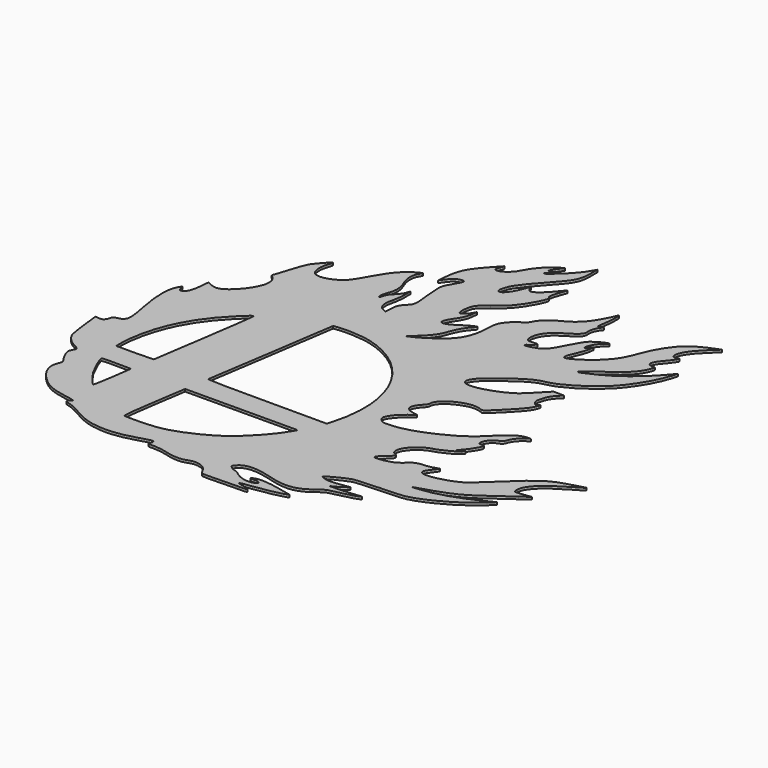
from build123d import *

# Parameters (mm, degrees)
F1_DEPTH = 0.4


# Not quite as in the source:
# - ends of sketch curves that miss each other by under 0.0002 mm in the source are joined


with BuildPart() as f1:
    # F0 (on Top) → F1 (new body)
    with BuildSketch(Plane.XY):
        with BuildLine():
            add(Edge.make_bspline(
                [(-1.4960361405, -38.6585897683), (-1.616879416, -38.6031296058), (-1.8647027683, -38.265785706), (-2.0467534003, -37.9089393314)],
                knots=[0, 0, 0, 0, 1, 1, 1, 1], degree=3))
            add(Edge.make_bspline(
                [(0.6166918414, -38.6753123078), (-0.4244712896, -38.7216066193), (-1.3752026214, -38.7140941599), (-1.4960361405, -38.6585897683)],
                knots=[0, 0, 0, 0, 1, 1, 1, 1], degree=3))
            add(Edge.make_bspline(
                [(4.3166854176, -38.5834606212), (3.3228507809, -38.5878510196), (1.6578504194, -38.6290231997), (0.6166918414, -38.6753123078)],
                knots=[0, 0, 0, 0, 1, 1, 1, 1], degree=3))
            add(Edge.make_bspline(
                [(5.6934265327, -38.3445448994), (6.0777086692, -38.5510887507), (5.9306739032, -38.5766063964), (4.3166854176, -38.5834606212)],
                knots=[0, 0, 0, 0, 1, 1, 1, 1], degree=3))
            add(Edge.make_bspline(
                [(4.5029020498, -37.9872393216), (4.9210631017, -38.0565737933), (5.4567990215, -38.2173599373), (5.6934265327, -38.3445448994)],
                knots=[0, 0, 0, 0, 1, 1, 1, 1], degree=3))
            add(Edge.make_bspline(
                [(5.8868336618, -37.4158195449), (3.8808118727, -37.6312027316), (3.4438156867, -37.811633144), (4.5029020498, -37.9872393216)],
                knots=[0, 0, 0, 0, 1, 1, 1, 1], degree=3))
            add(Edge.make_bspline(
                [(11.0283023377, -36.219943329), (11.677959013, -36.3096681115), (7.8099744864, -37.2093342322), (5.8868336618, -37.4158195449)],
                knots=[0, 0, 0, 0, 1, 1, 1, 1], degree=3))
            add(Edge.make_bspline(
                [(8.8203417373, -35.7401651502), (9.7980932067, -35.9713635274), (10.791674176, -36.1872638054), (11.0283023377, -36.219943329)],
                knots=[0, 0, 0, 0, 1, 1, 1, 1], degree=3))
            add(Edge.make_bspline(
                [(4.4887792766, -35.5779448093), (5.138255783, -35.2066686588), (6.8325007504, -35.2701193462), (8.8203417373, -35.7401651502)],
                knots=[0, 0, 0, 0, 1, 1, 1, 1], degree=3))
            add(Edge.make_bspline(
                [(4.865826687, -35.829982944), (4.0790868153, -35.8240315151), (4.069491681, -35.8176410464), (4.4887792766, -35.5779448093)],
                knots=[0, 0, 0, 0, 1, 1, 1, 1], degree=3))
            add(Edge.make_bspline(
                [(4.8935349788, -36.6414118144), (6.1954201273, -36.4667910373), (6.1740190492, -35.8398662185), (4.865826687, -35.829982944)],
                knots=[0, 0, 0, 0, 1, 1, 1, 1], degree=3))
            add(Edge.make_bspline(
                [(2.1650389935, -35.8356859089), (2.9463445277, -36.4565955566), (3.9849176489, -36.7632840692), (4.8935349788, -36.6414118144)],
                knots=[0, 0, 0, 0, 1, 1, 1, 1], degree=3))
            add(Edge.make_bspline(
                [(1.2144253893, -35.3198043461), (1.380226344, -35.3198043461), (1.8080020431, -35.5519536511), (2.1650389935, -35.8356859089)],
                knots=[0, 0, 0, 0, 1, 1, 1, 1], degree=3))
            add(Edge.make_bspline(
                [(0.5066931751, -34.9898610318), (0.7301449383, -35.1713308303), (1.0486244347, -35.3198043461), (1.2144253893, -35.3198043461)],
                knots=[0, 0, 0, 0, 1, 1, 1, 1], degree=3))
            Line((0.5066931751, -34.9898610318), (0.100420021, -34.6599177174))
            Line((0.100420021, -34.6599177174), (0.4610915708, -34.175212536))
            add(Edge.make_bspline(
                [(5.8655301481, -33.857894056), (3.1059013602, -33.0377533344), (1.2253233337, -33.1481715278), (0.4610915708, -34.175212536)],
                knots=[0, 0, 0, 0, 1, 1, 1, 1], degree=3))
            add(Edge.make_bspline(
                [(12.6137044518, -33.1117702472), (10.6733532656, -34.5919641074), (8.9694591782, -34.7803557754), (5.8655301481, -33.857894056)],
                knots=[0, 0, 0, 0, 1, 1, 1, 1], degree=3))
            add(Edge.make_bspline(
                [(15.9329574795, -31.704964985), (13.9335310444, -32.1195304633), (13.8905005875, -32.1377704546), (12.6137044518, -33.1117702472)],
                knots=[0, 0, 0, 0, 1, 1, 1, 1], degree=3))
            add(Edge.make_bspline(
                [(18.7724869644, -30.783088652), (18.7724869644, -30.9441577329), (17.3058987861, -31.4202961089), (15.9329574795, -31.704964985)],
                knots=[0, 0, 0, 0, 1, 1, 1, 1], degree=3))
            add(Edge.make_bspline(
                [(17.8690015223, -30.8601450213), (18.3659165642, -30.7860396502), (18.7724869644, -30.7513607066), (18.7724869644, -30.783088652)],
                knots=[0, 0, 0, 0, 1, 1, 1, 1], degree=3))
            add(Edge.make_bspline(
                [(15.2942182614, -31.0492098838), (16.2134310861, -31.0193063928), (17.372081277, -30.9342549455), (17.8690015223, -30.8601450213)],
                knots=[0, 0, 0, 0, 1, 1, 1, 1], degree=3))
            Line((15.2942182614, -31.0492098838), (13.6229204427, -31.1035291931))
            Line((13.6229204427, -31.1035291931), (14.2121457238, -30.8015868638))
            add(Edge.make_bspline(
                [(15.9139473798, -29.6420436333), (16.1085246314, -29.6400923452), (14.9872025829, -30.404416469), (14.2121457238, -30.8015868638)],
                knots=[0, 0, 0, 0, 1, 1, 1, 1], degree=3))
            add(Edge.make_bspline(
                [(14.6422584156, -29.8266745187), (15.2574898149, -29.7258417032), (15.8297538489, -29.6427558535), (15.9139473798, -29.6420436333)],
                knots=[0, 0, 0, 0, 1, 1, 1, 1], degree=3))
            add(Edge.make_bspline(
                [(11.6318943031, -29.7711551672), (12.1821328468, -30.0594579923), (13.1167510915, -30.0766930701), (14.6422584156, -29.8266745187)],
                knots=[0, 0, 0, 0, 1, 1, 1, 1], degree=3))
            Line((11.6318943031, -29.7711551672), (11.1691606263, -29.5287076138))
            Line((11.1691606263, -29.5287076138), (11.5721699256, -29.2646397876))
            add(Edge.make_bspline(
                [(14.7283056703, -27.7477181313), (14.0168412922, -27.9661700439), (12.2794975728, -28.8011847846), (11.5721699256, -29.2646397876)],
                knots=[0, 0, 0, 0, 1, 1, 1, 1], degree=3))
            add(Edge.make_bspline(
                [(19.2027167335, -27.4117453366), (17.0792664232, -27.4816307219), (15.1143875449, -27.6291728228), (14.7283056703, -27.7477181313)],
                knots=[0, 0, 0, 0, 1, 1, 1, 1], degree=3))
            add(Edge.make_bspline(
                [(24.3266921111, -26.8288565385), (23.1013364842, -27.2485740679), (22.670194813, -27.2976196958), (19.2027167335, -27.4117453366)],
                knots=[0, 0, 0, 0, 1, 1, 1, 1], degree=3))
            add(Edge.make_bspline(
                [(32.5339271738, -21.9328456033), (30.576633603, -23.8032918912), (27.0934671667, -25.8811698667), (24.3266921111, -26.8288565385)],
                knots=[0, 0, 0, 0, 1, 1, 1, 1], degree=3))
            Line((32.5339271738, -21.9328456033), (33.4864192179, -21.0226184605))
            Line((33.4864192179, -21.0226184605), (31.8519617196, -21.8269004128))
            add(Edge.make_bspline(
                [(23.0748041687, -24.5515764264), (25.7331656543, -24.3257343352), (28.5522846651, -23.45060111), (31.8519617196, -21.8269004128)],
                knots=[0, 0, 0, 0, 1, 1, 1, 1], degree=3))
            add(Edge.make_bspline(
                [(22.5585271449, -24.4671149186), (22.044635896, -24.6202572165), (22.1204388879, -24.6326576527), (23.0748041687, -24.5515764264)],
                knots=[0, 0, 0, 0, 1, 1, 1, 1], degree=3))
            add(Edge.make_bspline(
                [(28.3081004652, -22.3656946515), (27.1254832523, -22.9809605235), (25.2704228715, -23.6589694158), (22.5585271449, -24.4671149186)],
                knots=[0, 0, 0, 0, 1, 1, 1, 1], degree=3))
            add(Edge.make_bspline(
                [(34.690842076, -18.0392497692), (30.3756561263, -21.1638962761), (29.5751642261, -21.7064961771), (28.3081004652, -22.3656946515)],
                knots=[0, 0, 0, 0, 1, 1, 1, 1], degree=3))
            Line((34.690842076, -18.0392497692), (36.067363346, -17.0425077131))
            Line((36.067363346, -17.0425077131), (35.0350297939, -17.175888015))
            add(Edge.make_bspline(
                [(33.3276669666, -16.6251805117), (33.3126420477, -17.426233082), (33.2510743534, -17.406374172), (35.0350297939, -17.175888015)],
                knots=[0, 0, 0, 0, 1, 1, 1, 1], degree=3))
            add(Edge.make_bspline(
                [(38.3469069523, -11.653620252), (35.0399418366, -13.5346574816), (33.3543313192, -15.2042524762), (33.3276669666, -16.6251805117)],
                knots=[0, 0, 0, 0, 1, 1, 1, 1], degree=3))
            add(Edge.make_bspline(
                [(40.0602016956, -10.6013835607), (40.0874221654, -10.6286040305), (39.3164630114, -11.1021276804), (38.3469069523, -11.653620252)],
                knots=[0, 0, 0, 0, 1, 1, 1, 1], degree=3))
            add(Edge.make_bspline(
                [(35.957130525, -11.8125969015), (36.6965366991, -11.5013274148), (39.9883988445, -10.5295807095), (40.0602016956, -10.6013835607)],
                knots=[0, 0, 0, 0, 1, 1, 1, 1], degree=3))
            add(Edge.make_bspline(
                [(30.3121221839, -16.1104892347), (33.0413303895, -13.4712451696), (34.3080429185, -12.5068209983), (35.957130525, -11.8125969015)],
                knots=[0, 0, 0, 0, 1, 1, 1, 1], degree=3))
            add(Edge.make_bspline(
                [(26.5066224571, -19.4354699435), (27.0216792754, -19.1326788039), (28.7341544777, -17.6364408021), (30.3121221839, -16.1104892347)],
                knots=[0, 0, 0, 0, 1, 1, 1, 1], degree=3))
            add(Edge.make_bspline(
                [(20.699925176, -20.6574979737), (21.2540474336, -21.2116202314), (24.7294574995, -20.4802136883), (26.5066224571, -19.4354699435)],
                knots=[0, 0, 0, 0, 1, 1, 1, 1], degree=3))
            add(Edge.make_bspline(
                [(21.1857861705, -19.158537925), (20.448765121, -20.0909414576), (20.371557852, -20.3291306498), (20.699925176, -20.6574979737)],
                knots=[0, 0, 0, 0, 1, 1, 1, 1], degree=3))
            add(Edge.make_bspline(
                [(21.8097495842, -18.2826196315), (21.8473606634, -18.2826196315), (21.5665898106, -18.6767798391), (21.1857861705, -19.158537925)],
                knots=[0, 0, 0, 0, 1, 1, 1, 1], degree=3))
            add(Edge.make_bspline(
                [(21.0096921708, -18.5407555417), (21.4120965708, -18.3987798154), (21.7721241955, -18.2826196315), (21.8097495842, -18.2826196315)],
                knots=[0, 0, 0, 0, 1, 1, 1, 1], degree=3))
            add(Edge.make_bspline(
                [(19.6532008737, -18.7988960049), (19.9968662968, -18.7988960049), (20.6072877708, -18.6827358209), (21.0096921708, -18.5407555417)],
                knots=[0, 0, 0, 0, 1, 1, 1, 1], degree=3))
            add(Edge.make_bspline(
                [(17.3102891845, -19.7098698405), (17.9152763209, -19.0869354061), (18.656073113, -18.7988960049), (19.6532008737, -18.7988960049)],
                knots=[0, 0, 0, 0, 1, 1, 1, 1], degree=3))
            add(Edge.make_bspline(
                [(14.6314775486, -21.0381455108), (15.8226661199, -20.812244881), (16.6270209202, -20.4134067853), (17.3102891845, -19.7098698405)],
                knots=[0, 0, 0, 0, 1, 1, 1, 1], degree=3))
            add(Edge.make_bspline(
                [(13.8768168541, -20.0730286323), (12.6153871126, -21.1066747509), (12.829082435, -21.3799624136), (14.6314775486, -21.0381455108)],
                knots=[0, 0, 0, 0, 1, 1, 1, 1], degree=3))
            add(Edge.make_bspline(
                [(14.5631388843, -18.6294363849), (15.1236659201, -18.8425463209), (14.9610553216, -19.1845778654), (13.8768168541, -20.0730286323)],
                knots=[0, 0, 0, 0, 1, 1, 1, 1], degree=3))
            add(Edge.make_bspline(
                [(14.1259820422, -17.8825418174), (14.1259820422, -18.346046253), (14.2141997798, -18.4967683032), (14.5631388843, -18.6294363849)],
                knots=[0, 0, 0, 0, 1, 1, 1, 1], degree=3))
            add(Edge.make_bspline(
                [(17.5272236453, -14.5031351288), (15.8692186519, -14.9205403818), (14.1259820422, -16.6525863538), (14.1259820422, -17.8825418174)],
                knots=[0, 0, 0, 0, 1, 1, 1, 1], degree=3))
            add(Edge.make_bspline(
                [(20.9525974794, -12.7381904384), (20.5213582438, -13.2221925057), (18.5207851017, -14.2529995), (17.5272236453, -14.5031351288)],
                knots=[0, 0, 0, 0, 1, 1, 1, 1], degree=3))
            Line((20.9525974794, -12.7381904384), (21.2678332844, -12.3843828699))
            Line((21.2678332844, -12.3843828699), (20.6655096564, -12.6862224314))
            Line((20.6655096564, -12.6862224314), (20.0631808248, -12.9880671963))
            Line((20.0631808248, -12.9880671963), (20.605517302, -12.408602909))
            add(Edge.make_bspline(
                [(22.2143446304, -9.8324979756), (22.2143446304, -10.2079453297), (21.3102152632, -11.6556645515), (20.605517302, -12.408602909)],
                knots=[0, 0, 0, 0, 1, 1, 1, 1], degree=3))
            add(Edge.make_bspline(
                [(21.8525413335, -9.6327250941), (22.1160823119, -9.5638101495), (22.2143446304, -9.618090433), (22.2143446304, -9.8324979756)],
                knots=[0, 0, 0, 0, 1, 1, 1, 1], degree=3))
            add(Edge.make_bspline(
                [(22.0717880707, -7.8725604093), (21.1689270408, -8.6322703871), (21.0170927564, -9.8512010726), (21.8525413335, -9.6327250941)],
                knots=[0, 0, 0, 0, 1, 1, 1, 1], degree=3))
            add(Edge.make_bspline(
                [(22.9941866985, -7.3379907095), (22.7691641483, -7.3944707451), (22.3540861317, -7.635025549), (22.0717880707, -7.8725604093)],
                knots=[0, 0, 0, 0, 1, 1, 1, 1], degree=3))
            add(Edge.make_bspline(
                [(23.5980368844, -6.6452977234), (23.4692375566, -7.0355651111), (23.2648056495, -7.2700709217), (22.9941866985, -7.3379907095)],
                knots=[0, 0, 0, 0, 1, 1, 1, 1], degree=3))
            add(Edge.make_bspline(
                [(25.2186304804, -4.6637015091), (24.5170110014, -5.0915650161), (23.835991922, -5.9242869932), (23.5980368844, -6.6452977234)],
                knots=[0, 0, 0, 0, 1, 1, 1, 1], degree=3))
            Line((25.2186304804, -4.6637015091), (25.7422443477, -4.3443972682))
            Line((25.7422443477, -4.3443972682), (25.2259673238, -4.3453729122))
            add(Edge.make_bspline(
                [(21.2785458564, -6.8326604122), (22.9065198747, -5.1467572016), (24.1749892134, -4.3474855069), (25.2259673238, -4.3453729122)],
                knots=[0, 0, 0, 0, 1, 1, 1, 1], degree=3))
            add(Edge.make_bspline(
                [(15.6169125403, -10.8041711823), (18.0962680538, -9.6310905651), (19.5840862473, -8.5874200288), (21.2785458564, -6.8326604122)],
                knots=[0, 0, 0, 0, 1, 1, 1, 1], degree=3))
            add(Edge.make_bspline(
                [(9.2795429321, -12.7348387758), (10.9906958115, -12.6352404753), (13.1140927866, -11.9883539787), (15.6169125403, -10.8041711823)],
                knots=[0, 0, 0, 0, 1, 1, 1, 1], degree=3))
            add(Edge.make_bspline(
                [(7.3328110337, -12.365504157), (7.7724902409, -12.8051827138), (7.8425805115, -12.8184807426), (9.2795429321, -12.7348387758)],
                knots=[0, 0, 0, 0, 1, 1, 1, 1], degree=3))
            add(Edge.make_bspline(
                [(6.9906624119, -11.5250596318), (6.9067524682, -11.808069913), (6.9969553162, -12.0296529926), (7.3328110337, -12.365504157)],
                knots=[0, 0, 0, 0, 1, 1, 1, 1], degree=3))
            add(Edge.make_bspline(
                [(8.9962991468, -9.0781247709), (7.9928687253, -9.8324147206), (7.2089387085, -10.7888340574), (6.9906624119, -11.5250596318)],
                knots=[0, 0, 0, 0, 1, 1, 1, 1], degree=3))
            Line((8.9962991468, -9.0781247709), (10.0064419996, -8.3187861883))
            Line((10.0064419996, -8.3187861883), (9.3557504911, -8.2046208713))
            add(Edge.make_bspline(
                [(7.930642146, -7.2561146584), (7.930642146, -7.6820854159), (8.4866369898, -8.0521374583), (9.3557504911, -8.2046208713)],
                knots=[0, 0, 0, 0, 1, 1, 1, 1], degree=3))
            add(Edge.make_bspline(
                [(8.8608016972, -5.5607229839), (8.3241239557, -6.0620967193), (7.930642146, -6.7792926811), (7.930642146, -7.2561146584)],
                knots=[0, 0, 0, 0, 1, 1, 1, 1], degree=3))
            add(Edge.make_bspline(
                [(9.3080271862, -4.7863054969), (9.3076857108, -4.9827709449), (9.1064200939, -5.3312612532), (8.8608016972, -5.5607229839)],
                knots=[0, 0, 0, 0, 1, 1, 1, 1], degree=3))
            add(Edge.make_bspline(
                [(12.7867980207, -1.9114973726), (10.776752025, -2.5236990717), (9.3099199357, -3.7358737472), (9.3080271862, -4.7863054969)],
                knots=[0, 0, 0, 0, 1, 1, 1, 1], degree=3))
            add(Edge.make_bspline(
                [(15.6837682255, -2.0041198179), (14.7023873602, -1.5911394361), (13.9206818119, -1.5661434348), (12.7867980207, -1.9114973726)],
                knots=[0, 0, 0, 0, 1, 1, 1, 1], degree=3))
            add(Edge.make_bspline(
                [(18.0237191602, -0.0023765533), (16.5543699092, -1.5009853703), (15.8730919589, -2.0837909133), (15.6837682255, -2.0041198179)],
                knots=[0, 0, 0, 0, 1, 1, 1, 1], degree=3))
            add(Edge.make_bspline(
                [(20.7447950471, 3.5410456612), (20.4586483955, 2.614179234), (19.987037008, 2.0000353526), (18.0237191602, -0.0023765533)],
                knots=[0, 0, 0, 0, 1, 1, 1, 1], degree=3))
            add(Edge.make_bspline(
                [(20.4979766083, 3.7131395201), (20.8421012345, 3.9234688705), (20.8591795589, 3.9115614597), (20.7447950471, 3.5410456612)],
                knots=[0, 0, 0, 0, 1, 1, 1, 1], degree=3))
            add(Edge.make_bspline(
                [(19.8806085485, 3.8212265746), (20.0959624659, 3.5307428597), (20.1764875751, 3.5166448028), (20.4979766083, 3.7131395201)],
                knots=[0, 0, 0, 0, 1, 1, 1, 1], degree=3))
            add(Edge.make_bspline(
                [(19.9005604699, 5.6165775378), (19.569871113, 4.5030209658), (19.566992963, 4.2442365775), (19.8806085485, 3.8212265746)],
                knots=[0, 0, 0, 0, 1, 1, 1, 1], degree=3))
            add(Edge.make_bspline(
                [(20.8470718159, 7.1966526353), (20.3994170435, 6.7489926595), (20.0770349707, 6.2108176295), (19.9005604699, 5.6165775378)],
                knots=[0, 0, 0, 0, 1, 1, 1, 1], degree=3))
            Line((20.8470718159, 7.1966526353), (21.5259594382, 7.8755396072))
            Line((21.5259594382, 7.8755396072), (20.6394306901, 7.8755396072))
            Line((20.6394306901, 7.8755396072), (19.7528967387, 7.8755396072))
            Line((19.7528967387, 7.8755396072), (18.0924090563, 6.1631723762))
            add(Edge.make_bspline(
                [(14.9777876175, 3.7556242667), (16.2268897709, 4.3527867377), (16.6660518868, 4.6922523382), (18.0924090563, 6.1631723762)],
                knots=[0, 0, 0, 0, 1, 1, 1, 1], degree=3))
            add(Edge.make_bspline(
                [(9.2336193654, 2.6389996193), (9.8188549127, 2.0537692755), (12.5137692289, 2.5776413632), (14.9777876175, 3.7556242667)],
                knots=[0, 0, 0, 0, 1, 1, 1, 1], degree=3))
            add(Edge.make_bspline(
                [(9.3942689193, 4.0990848046), (8.8962761159, 3.4143439682), (8.8528645074, 3.0197590302), (9.2336193654, 2.6389996193)],
                knots=[0, 0, 0, 0, 1, 1, 1, 1], degree=3))
            add(Edge.make_bspline(
                [(12.7497820844, 6.9913673648), (10.2375571218, 5.0959003592), (9.9204142578, 4.8225398484), (9.3942689193, 4.0990848046)],
                knots=[0, 0, 0, 0, 1, 1, 1, 1], degree=3))
            add(Edge.make_bspline(
                [(17.6210558893, 9.4851767202), (15.9040543489, 9.1252616198), (14.8898625732, 8.6060531107), (12.7497820844, 6.9913673648)],
                knots=[0, 0, 0, 0, 1, 1, 1, 1], degree=3))
            add(Edge.make_bspline(
                [(24.4886197588, 13.6936031418), (22.4831001012, 11.7662377783), (19.3532488584, 9.8482724203), (17.6210558893, 9.4851767202)],
                knots=[0, 0, 0, 0, 1, 1, 1, 1], degree=3))
            add(Edge.make_bspline(
                [(29.0030517421, 21.0406368867), (28.2890754057, 18.6165080313), (26.3825445963, 15.5137159518), (24.4886197588, 13.6936031418)],
                knots=[0, 0, 0, 0, 1, 1, 1, 1], degree=3))
            Line((29.0030517421, 21.0406368867), (29.2564850478, 21.9011016284))
            Line((29.2564850478, 21.9011016284), (28.4581102952, 20.9545902824))
            add(Edge.make_bspline(
                [(21.2674527832, 15.184914141), (23.7298516028, 16.3667508386), (26.3860035797, 18.4980063016), (28.4581102952, 20.9545902824)],
                knots=[0, 0, 0, 0, 1, 1, 1, 1], degree=3))
            add(Edge.make_bspline(
                [(18.772477208, 14.2324168934), (18.772477208, 14.0389323633), (19.2969099659, 14.2391488376), (21.2674527832, 15.184914141)],
                knots=[0, 0, 0, 0, 1, 1, 1, 1], degree=3))
            add(Edge.make_bspline(
                [(22.2515504921, 16.983694168), (20.4812592722, 15.7729543398), (18.772477208, 14.4216385094), (18.772477208, 14.2324168934)],
                knots=[0, 0, 0, 0, 1, 1, 1, 1], degree=3))
            add(Edge.make_bspline(
                [(25.7400146757, 21.1096929745), (25.2685541878, 19.587454058), (24.1852868114, 18.3062187417), (22.2515504921, 16.983694168)],
                knots=[0, 0, 0, 0, 1, 1, 1, 1], degree=3))
            add(Edge.make_bspline(
                [(25.6330255461, 21.4334656653), (25.8107443184, 21.5011311351), (25.8368135282, 21.4222457584), (25.7400146757, 21.1096929745)],
                knots=[0, 0, 0, 0, 1, 1, 1, 1], degree=3))
            add(Edge.make_bspline(
                [(25.0108378046, 21.4879358742), (25.2238065974, 21.4087721137), (25.5037871785, 21.384258731), (25.6330255461, 21.4334656653)],
                knots=[0, 0, 0, 0, 1, 1, 1, 1], degree=3))
            add(Edge.make_bspline(
                [(25.4554973497, 23.4503951551), (24.5264649926, 22.3616882378), (24.381494039, 21.7218758112), (25.0108378046, 21.4879358742)],
                knots=[0, 0, 0, 0, 1, 1, 1, 1], degree=3))
            add(Edge.make_bspline(
                [(26.5834004426, 24.9263982988), (26.4205752024, 24.6507593338), (25.9130210871, 23.9865603583), (25.4554973497, 23.4503951551)],
                knots=[0, 0, 0, 0, 1, 1, 1, 1], degree=3))
            add(Edge.make_bspline(
                [(26.4829338189, 25.2808933711), (26.8783376475, 25.4271476219), (26.8786205842, 25.4261622214), (26.5834004426, 24.9263982988)],
                knots=[0, 0, 0, 0, 1, 1, 1, 1], degree=3))
            add(Edge.make_bspline(
                [(25.6578023527, 25.8305517319), (25.6558510645, 25.2217160048), (25.8941079014, 25.0631003436), (26.4829338189, 25.2808933711)],
                knots=[0, 0, 0, 0, 1, 1, 1, 1], degree=3))
            add(Edge.make_bspline(
                [(28.0709259428, 29.4469911492), (26.5390476628, 28.0059063071), (25.6603487837, 26.6890359161), (25.6578023527, 25.8305517319)],
                knots=[0, 0, 0, 0, 1, 1, 1, 1], degree=3))
            Line((28.0709259428, 29.4469911492), (29.4821951019, 30.774608585))
            Line((29.4821951019, 30.774608585), (28.558723916, 30.4111909223))
            add(Edge.make_bspline(
                [(24.4790291775, 27.8889708114), (25.2907500906, 28.823193595), (26.6344708571, 29.6539350146), (28.558723916, 30.4111909223)],
                knots=[0, 0, 0, 0, 1, 1, 1, 1], degree=3))
            add(Edge.make_bspline(
                [(21.8719078684, 23.4639468514), (22.4824906488, 25.105936322), (23.3705069289, 26.6131503197), (24.4790291775, 27.8889708114)],
                knots=[0, 0, 0, 0, 1, 1, 1, 1], degree=3))
            add(Edge.make_bspline(
                [(19.209902027, 18.9618515622), (20.4809906449, 20.2397306629), (20.9983064044, 21.11463949), (21.8719078684, 23.4639468514)],
                knots=[0, 0, 0, 0, 1, 1, 1, 1], degree=3))
            add(Edge.make_bspline(
                [(15.2007027765, 16.2267654263), (16.1328376818, 16.5018092484), (18.0931895716, 17.8391681651), (19.209902027, 18.9618515622)],
                knots=[0, 0, 0, 0, 1, 1, 1, 1], degree=3))
            add(Edge.make_bspline(
                [(15.2180204589, 17.9838659383), (14.5602217085, 16.5456007076), (14.555211451, 16.0362949859), (15.2007027765, 16.2267654263)],
                knots=[0, 0, 0, 0, 1, 1, 1, 1], degree=3))
            add(Edge.make_bspline(
                [(15.9448265149, 20.0849304205), (15.8811019967, 19.664057078), (15.5540420359, 18.7185799148), (15.2180204589, 17.9838659383)],
                knots=[0, 0, 0, 0, 1, 1, 1, 1], degree=3))
            Line((15.9448265149, 20.0849304205), (16.0606888022, 20.8501475838))
            Line((16.0606888022, 20.8501475838), (15.6150536131, 20.3430663307))
            add(Edge.make_bspline(
                [(15.167759829, 20.1801727954), (15.1692232951, 19.8774935296), (15.2231621032, 19.8971384483), (15.6150536131, 20.3430663307)],
                knots=[0, 0, 0, 0, 1, 1, 1, 1], degree=3))
            add(Edge.make_bspline(
                [(16.4351897816, 22.41832958), (15.8016650559, 21.9351171339), (15.1647255759, 20.8103413054), (15.167759829, 20.1801727954)],
                knots=[0, 0, 0, 0, 1, 1, 1, 1], degree=3))
            add(Edge.make_bspline(
                [(16.9812239498, 22.9753150277), (17.0250791511, 22.9314598264), (16.7793482302, 22.6808311722), (16.4351897816, 22.41832958)],
                knots=[0, 0, 0, 0, 1, 1, 1, 1], degree=3))
            add(Edge.make_bspline(
                [(14.5015022445, 21.6478146692), (15.0475019399, 22.1938189177), (16.8159791123, 23.1405598652), (16.9812239498, 22.9753150277)],
                knots=[0, 0, 0, 0, 1, 1, 1, 1], degree=3))
            add(Edge.make_bspline(
                [(12.9156513341, 19.0502254028), (13.4749737747, 20.1660064434), (14.1886086356, 21.3349204099), (14.5015022445, 21.6478146692)],
                knots=[0, 0, 0, 0, 1, 1, 1, 1], degree=3))
            add(Edge.make_bspline(
                [(9.7678820626, 15.8772454883), (11.3381616935, 16.3305934691), (11.7711135096, 16.7670231312), (12.9156513341, 19.0502254028)],
                knots=[0, 0, 0, 0, 1, 1, 1, 1], degree=3))
            add(Edge.make_bspline(
                [(8.8774266723, 16.0672866453), (8.3058260763, 15.656199013), (8.7062499188, 15.5707423482), (9.7678820626, 15.8772454883)],
                knots=[0, 0, 0, 0, 1, 1, 1, 1], degree=3))
            add(Edge.make_bspline(
                [(8.9671273889, 17.0357207137), (10.0982741732, 17.144412017), (10.0785173806, 16.9310776829), (8.8774266723, 16.0672866453)],
                knots=[0, 0, 0, 0, 1, 1, 1, 1], degree=3))
            add(Edge.make_bspline(
                [(7.947530545, 17.3822837997), (8.0978135554, 16.9870016015), (8.1776602667, 16.9598643866), (8.9671273889, 17.0357207137)],
                knots=[0, 0, 0, 0, 1, 1, 1, 1], degree=3))
            add(Edge.make_bspline(
                [(7.9163099345, 18.3933340015), (7.8438046196, 18.073127615), (7.8578538943, 17.618155512), (7.947530545, 17.3822837997)],
                knots=[0, 0, 0, 0, 1, 1, 1, 1], degree=3))
            add(Edge.make_bspline(
                [(11.0706160214, 21.8866133138), (9.0837701914, 20.7325532031), (8.2325356931, 19.7898416656), (7.9163099345, 18.3933340015)],
                knots=[0, 0, 0, 0, 1, 1, 1, 1], degree=3))
            add(Edge.make_bspline(
                [(12.6952780532, 23.856116745), (12.8234386593, 23.1856931603), (12.3784669081, 22.6462790624), (11.0706160214, 21.8866133138)],
                knots=[0, 0, 0, 0, 1, 1, 1, 1], degree=3))
            add(Edge.make_bspline(
                [(13.4011610967, 25.8342884487), (12.9427157008, 25.317894998), (12.5996356642, 24.3564413378), (12.6952780532, 23.856116745)],
                knots=[0, 0, 0, 0, 1, 1, 1, 1], degree=3))
            add(Edge.make_bspline(
                [(13.3163776263, 25.9331504631), (13.6826194534, 26.1580611395), (13.6855567925, 26.1546366287), (13.4011610967, 25.8342884487)],
                knots=[0, 0, 0, 0, 1, 1, 1, 1], degree=3))
            add(Edge.make_bspline(
                [(12.8238237135, 25.8133413703), (12.8860652526, 25.7510952781), (13.1077166273, 25.8049996135), (13.3163776263, 25.9331504631)],
                knots=[0, 0, 0, 0, 1, 1, 1, 1], degree=3))
            add(Edge.make_bspline(
                [(12.9020410992, 27.0255745844), (12.7967736562, 26.4210895795), (12.7615776213, 25.8755874625), (12.8238237135, 25.8133413703)],
                knots=[0, 0, 0, 0, 1, 1, 1, 1], degree=3))
            add(Edge.make_bspline(
                [(13.0817892112, 29.1430929787), (13.0881796799, 28.5829412407), (13.0073085422, 27.6300543859), (12.9020410992, 27.0255745844)],
                knots=[0, 0, 0, 0, 1, 1, 1, 1], degree=3))
            add(Edge.make_bspline(
                [(12.8834160538, 29.7313231029), (13.0460461651, 30.106038724), (13.0716425127, 30.0301433712), (13.0817892112, 29.1430929787)],
                knots=[0, 0, 0, 0, 1, 1, 1, 1], degree=3))
            add(Edge.make_bspline(
                [(8.1919144267, 24.0561478469), (10.2905150824, 25.0921647806), (11.5104409248, 26.567875231), (12.8834160538, 29.7313231029)],
                knots=[0, 0, 0, 0, 1, 1, 1, 1], degree=3))
            add(Edge.make_bspline(
                [(5.257357859, 21.4593052735), (5.7911034648, 22.5126060672), (6.7069743833, 23.323078156), (8.1919144267, 24.0561478469)],
                knots=[0, 0, 0, 0, 1, 1, 1, 1], degree=3))
            add(Edge.make_bspline(
                [(4.3949418291, 20.5377756193), (4.708742787, 20.6165341623), (4.9738259335, 20.8997883545), (5.257357859, 21.4593052735)],
                knots=[0, 0, 0, 0, 1, 1, 1, 1], degree=3))
            add(Edge.make_bspline(
                [(2.1177592814, 18.0950945666), (2.3625191113, 18.9192939675), (3.711410141, 20.3662183646), (4.3949418291, 20.5377756193)],
                knots=[0, 0, 0, 0, 1, 1, 1, 1], degree=3))
            add(Edge.make_bspline(
                [(1.9074052147, 16.5348393534), (1.9074052147, 17.003392422), (2.0020622032, 17.7055049264), (2.1177592814, 18.0950945666)],
                knots=[0, 0, 0, 0, 1, 1, 1, 1], degree=3))
            add(Edge.make_bspline(
                [(0.0097000817, 11.3173972732), (1.2509723661, 12.5316838928), (1.9074052147, 14.3364498215), (1.9074052147, 16.5348393534)],
                knots=[0, 0, 0, 0, 1, 1, 1, 1], degree=3))
            add(Edge.make_bspline(
                [(-4.2289856159, 8.3887531086), (-3.1583092515, 8.8367148836), (-1.0058530427, 10.3239138683), (0.0097000817, 11.3173972732)],
                knots=[0, 0, 0, 0, 1, 1, 1, 1], degree=3))
            Line((-4.2289856159, 8.3887531086), (-5.0623521685, 8.0400774279))
            Line((-5.0623521685, 8.0400774279), (-3.8953842866, 9.0961926297))
            add(Edge.make_bspline(
                [(-1.5388233367, 12.2639040661), (-1.8568585899, 11.2572345063), (-2.5767083036, 10.2896050191), (-3.8953842866, 9.0961926297)],
                knots=[0, 0, 0, 0, 1, 1, 1, 1], degree=3))
            add(Edge.make_bspline(
                [(0.1469627966, 15.3185526634), (-0.5026795693, 14.6484510412), (-1.1641467414, 13.4498625348), (-1.5388233367, 12.2639040661)],
                knots=[0, 0, 0, 0, 1, 1, 1, 1], degree=3))
            add(Edge.make_bspline(
                [(0.6461075104, 15.9639021953), (0.7156806896, 15.9639021953), (0.4910679099, 15.673491979), (0.1469627966, 15.3185526634)],
                knots=[0, 0, 0, 0, 1, 1, 1, 1], degree=3))
            add(Edge.make_bspline(
                [(-1.8113688595, 14.6792521248), (-0.7545856668, 15.4028483118), (0.3186813578, 15.9639021953), (0.6461075104, 15.9639021953)],
                knots=[0, 0, 0, 0, 1, 1, 1, 1], degree=3))
            add(Edge.make_bspline(
                [(-3.3758876374, 15.5087837458), (-4.5217868106, 13.8181636213), (-3.7029963804, 13.3840260724), (-1.8113688595, 14.6792521248)],
                knots=[0, 0, 0, 0, 1, 1, 1, 1], degree=3))
            add(Edge.make_bspline(
                [(-2.1187169075, 18.3272100493), (-2.228856717, 17.4082899178), (-2.4992031381, 16.8022146131), (-3.3758876374, 15.5087837458)],
                knots=[0, 0, 0, 0, 1, 1, 1, 1], degree=3))
            Line((-2.1187169075, 18.3272100493), (-2.0203765374, 19.1476141947))
            Line((-2.0203765374, 19.1476141947), (-2.2988546266, 18.6313378213))
            add(Edge.make_bspline(
                [(-3.5325806293, 17.5127326164), (-3.1925101294, 17.5127326164), (-2.6243633134, 18.0278629332), (-2.2988546266, 18.6313378213)],
                knots=[0, 0, 0, 0, 1, 1, 1, 1], degree=3))
            add(Edge.make_bspline(
                [(-3.4984818688, 19.9093970909), (-3.8477383829, 19.03652736), (-3.8694119909, 17.5127326164), (-3.5325806293, 17.5127326164)],
                knots=[0, 0, 0, 0, 1, 1, 1, 1], degree=3))
            add(Edge.make_bspline(
                [(-1.7796799399, 21.6424291139), (-2.8893684083, 20.8361861171), (-3.2888016469, 20.4334499981), (-3.4984818688, 19.9093970909)],
                knots=[0, 0, 0, 0, 1, 1, 1, 1], degree=3))
            add(Edge.make_bspline(
                [(0.3994796473, 23.5430618297), (-0.0039543824, 23.0753965973), (-0.9845742454, 22.2201125256), (-1.7796799399, 21.6424291139)],
                knots=[0, 0, 0, 0, 1, 1, 1, 1], degree=3))
            add(Edge.make_bspline(
                [(2.8031934755, 28.1420333724), (3.2700294105, 27.9864181419), (1.7903480887, 25.1553767605), (0.3994796473, 23.5430618297)],
                knots=[0, 0, 0, 0, 1, 1, 1, 1], degree=3))
            add(Edge.make_bspline(
                [(3.0183080349, 30.1576262298), (2.5553356505, 28.9276265371), (2.4828895247, 28.2488026568), (2.8031934755, 28.1420333724)],
                knots=[0, 0, 0, 0, 1, 1, 1, 1], degree=3))
            add(Edge.make_bspline(
                [(3.3925410374, 31.280158077), (3.4190785563, 31.280158077), (3.2506921448, 30.7750183555), (3.0183080349, 30.1576262298)],
                knots=[0, 0, 0, 0, 1, 1, 1, 1], degree=3))
            add(Edge.make_bspline(
                [(2.4144819149, 30.1341958121), (2.925856002, 30.764471643), (3.3659840056, 31.280158077), (3.3925410374, 31.280158077)],
                knots=[0, 0, 0, 0, 1, 1, 1, 1], degree=3))
            add(Edge.make_bspline(
                [(-0.1918244061, 28.0103942699), (0.3255011099, 28.0103942699), (1.4051442937, 28.8901618045), (2.4144819149, 30.1341958121)],
                knots=[0, 0, 0, 0, 1, 1, 1, 1], degree=3))
            add(Edge.make_bspline(
                [(-0.7383314365, 28.5332224185), (-0.6031312332, 28.2116696432), (-0.3927387911, 28.0103942699), (-0.1918244061, 28.0103942699)],
                knots=[0, 0, 0, 0, 1, 1, 1, 1], degree=3))
            Line((-0.7383314365, 28.5332224185), (-0.9581635602, 29.0560505671))
            Line((-0.9581635602, 29.0560505671), (-1.4614202886, 27.8028357487))
            add(Edge.make_bspline(
                [(-3.2731958947, 25.4290013456), (-2.772056314, 25.4290013456), (-2.0178639287, 26.4171577339), (-1.4614202886, 27.8028357487)],
                knots=[0, 0, 0, 0, 1, 1, 1, 1], degree=3))
            add(Edge.make_bspline(
                [(-3.2385117477, 27.3055499621), (-3.7583791418, 26.1167178964), (-3.7710963371, 25.4290013456), (-3.2731958947, 25.4290013456)],
                knots=[0, 0, 0, 0, 1, 1, 1, 1], degree=3))
            add(Edge.make_bspline(
                [(0.5130979532, 32.0398101665), (-1.7527911891, 29.5660737124), (-2.8622155832, 28.1660582826), (-3.2385117477, 27.3055499621)],
                knots=[0, 0, 0, 0, 1, 1, 1, 1], degree=3))
            add(Edge.make_bspline(
                [(2.7678602, 36.9187349723), (2.7678602, 34.9134989019), (2.3834759461, 34.0817584227), (0.5130979532, 32.0398101665)],
                knots=[0, 0, 0, 0, 1, 1, 1, 1], degree=3))
            Line((2.7678602, 36.9187349723), (2.7678602, 38.2420829896))
            Line((2.7678602, 38.2420829896), (2.1225106681, 37.1493356049))
            add(Edge.make_bspline(
                [(0.0458034655, 34.7007792235), (0.8759497423, 35.4871073735), (1.7482295338, 36.5155754237), (2.1225106681, 37.1493356049)],
                knots=[0, 0, 0, 0, 1, 1, 1, 1], degree=3))
            add(Edge.make_bspline(
                [(-1.4658347528, 33.8325314438), (-2.7447239703, 32.4135625017), (-1.7898363947, 32.9620240724), (0.0458034655, 34.7007792235)],
                knots=[0, 0, 0, 0, 1, 1, 1, 1], degree=3))
            Line((-1.4658347528, 33.8325314438), (-1.1042272351, 34.2337462085))
            Line((-1.1042272351, 34.2337462085), (-1.5960103892, 34.1103870721))
            add(Edge.make_bspline(
                [(-1.8755811997, 34.3975431902), (-2.0800027, 34.002099035), (-2.0697389243, 33.9915568755), (-1.5960103892, 34.1103870721)],
                knots=[0, 0, 0, 0, 1, 1, 1, 1], degree=3))
            add(Edge.make_bspline(
                [(-1.2321244173, 35.3855116043), (-1.4693086962, 35.0679121389), (-1.7588596952, 34.6233267427), (-1.8755811997, 34.3975431902)],
                knots=[0, 0, 0, 0, 1, 1, 1, 1], degree=3))
            Line((-1.2321244173, 35.3855116043), (-0.8008845314, 35.962964764))
            Line((-0.8008845314, 35.962964764), (-1.2106940699, 35.7491751293))
            add(Edge.make_bspline(
                [(-4.9584116014, 31.6650587718), (-4.0055338526, 33.5472622214), (-2.6960295744, 34.9743062443), (-1.2106940699, 35.7491751293)],
                knots=[0, 0, 0, 0, 1, 1, 1, 1], degree=3))
            add(Edge.make_bspline(
                [(-7.6390717577, 30.0679300663), (-7.2696733968, 29.4702309912), (-5.5512272528, 30.4940770902), (-4.9584116014, 31.6650587718)],
                knots=[0, 0, 0, 0, 1, 1, 1, 1], degree=3))
            add(Edge.make_bspline(
                [(-7.4859197033, 30.8423475533), (-7.6260761785, 30.5069016064), (-7.6949956762, 30.1584158511), (-7.6390717577, 30.0679300663)],
                knots=[0, 0, 0, 0, 1, 1, 1, 1], degree=3))
            add(Edge.make_bspline(
                [(-7.2985862838, 31.4522467325), (-7.2614630267, 31.4522467325), (-7.345758675, 31.1777935003), (-7.4859197033, 30.8423475533)],
                knots=[0, 0, 0, 0, 1, 1, 1, 1], degree=3))
            add(Edge.make_bspline(
                [(-8.77003382, 29.8632789645), (-7.9978648674, 30.7372121475), (-7.3357147444, 31.4522467325), (-7.2985862838, 31.4522467325)],
                knots=[0, 0, 0, 0, 1, 1, 1, 1], degree=3))
            add(Edge.make_bspline(
                [(-11.4215508372, 24.1435512469), (-11.1869474622, 26.6645225334), (-10.7350928673, 27.6392449531), (-8.77003382, 29.8632789645)],
                knots=[0, 0, 0, 0, 1, 1, 1, 1], degree=3))
            Line((-11.4215508372, 24.1435512469), (-11.5331697232, 22.944142549))
            Line((-11.5331697232, 22.944142549), (-11.0116437342, 23.6640904776))
            add(Edge.make_bspline(
                [(-9.1925898233, 24.9445160093), (-9.8929708847, 24.870917973), (-10.3917396503, 24.519837655), (-11.0116437342, 23.6640904776)],
                knots=[0, 0, 0, 0, 1, 1, 1, 1], degree=3))
            add(Edge.make_bspline(
                [(-9.4632868258, 23.1814491086), (-8.5651192943, 24.6818479071), (-8.5138342381, 25.0158453479), (-9.1925898233, 24.9445160093)],
                knots=[0, 0, 0, 0, 1, 1, 1, 1], degree=3))
            add(Edge.make_bspline(
                [(-10.1329058294, 20.9442432517), (-10.1384182184, 21.9330097427), (-10.0662355165, 22.1742234316), (-9.4632868258, 23.1814491086)],
                knots=[0, 0, 0, 0, 1, 1, 1, 1], degree=3))
            add(Edge.make_bspline(
                [(-9.91779127, 18.2011028487), (-10.0326974261, 19.1002909039), (-10.1295008315, 20.3346998575), (-10.1329058294, 20.9442432517)],
                knots=[0, 0, 0, 0, 1, 1, 1, 1], degree=3))
            add(Edge.make_bspline(
                [(-10.4002667795, 15.0483727523), (-9.7007930672, 15.727694211), (-9.6468009239, 16.080516379), (-9.91779127, 18.2011028487)],
                knots=[0, 0, 0, 0, 1, 1, 1, 1], degree=3))
            add(Edge.make_bspline(
                [(-11.3437484254, 12.6829334413), (-11.3437484254, 13.7828596151), (-11.1163895329, 14.3528796677), (-10.4002667795, 15.0483727523)],
                knots=[0, 0, 0, 0, 1, 1, 1, 1], degree=3))
            add(Edge.make_bspline(
                [(-11.4383423222, 11.833674297), (-11.3863157766, 11.833674297), (-11.3437484254, 12.2158438389), (-11.3437484254, 12.6829334413)],
                knots=[0, 0, 0, 0, 1, 1, 1, 1], degree=3))
            add(Edge.make_bspline(
                [(-12.0343437767, 12.0929614672), (-11.7585682216, 11.9503561253), (-11.4903682175, 11.833674297), (-11.4383423222, 11.833674297)],
                knots=[0, 0, 0, 0, 1, 1, 1, 1], degree=3))
            add(Edge.make_bspline(
                [(-12.655819298, 14.8735418865), (-13.0185540099, 13.4968840263), (-12.7923847527, 12.4849602979), (-12.0343437767, 12.0929614672)],
                knots=[0, 0, 0, 0, 1, 1, 1, 1], degree=3))
            add(Edge.make_bspline(
                [(-12.3838585113, 17.1107470929), (-12.3799559349, 16.4637246566), (-12.5020870606, 15.4569868017), (-12.655819298, 14.8735418865)],
                knots=[0, 0, 0, 0, 1, 1, 1, 1], degree=3))
            Line((-12.3838585113, 17.1107470929), (-12.3914197529, 18.287149453))
            Line((-12.3914197529, 18.287149453), (-12.6342718734, 17.5987792207))
            add(Edge.make_bspline(
                [(-13.4944192055, 16.3880732148), (-13.1549048228, 16.6753561666), (-12.7678375477, 17.2201753327), (-12.6342718734, 17.5987792207)],
                knots=[0, 0, 0, 0, 1, 1, 1, 1], degree=3))
            add(Edge.make_bspline(
                [(-14.3436250146, 15.0973793543), (-14.1956243609, 15.5877478245), (-13.8883797313, 16.0547196991), (-13.4944192055, 16.3880732148)],
                knots=[0, 0, 0, 0, 1, 1, 1, 1], degree=3))
            add(Edge.make_bspline(
                [(-14.6909881287, 14.7694647292), (-14.5839066382, 14.360991823), (-14.5586907917, 14.3847975386), (-14.3436250146, 15.0973793543)],
                knots=[0, 0, 0, 0, 1, 1, 1, 1], degree=3))
            add(Edge.make_bspline(
                [(-14.4518480087, 16.1095560998), (-14.677602292, 15.5368042437), (-14.764498357, 15.0498700407), (-14.6909881287, 14.7694647292)],
                knots=[0, 0, 0, 0, 1, 1, 1, 1], degree=3))
            add(Edge.make_bspline(
                [(-14.5522612973, 19.5643462532), (-14.0049399293, 18.2025955842), (-13.9789728369, 17.3092373276), (-14.4518480087, 16.1095560998)],
                knots=[0, 0, 0, 0, 1, 1, 1, 1], degree=3))
            add(Edge.make_bspline(
                [(-14.634835259, 22.7640828814), (-15.1221987454, 21.9380590261), (-15.0958413954, 20.9167938308), (-14.5522612973, 19.5643462532)],
                knots=[0, 0, 0, 0, 1, 1, 1, 1], degree=3))
            add(Edge.make_bspline(
                [(-14.3395077966, 23.3638893477), (-14.307311542, 23.3638893477), (-14.440189062, 23.0939774135), (-14.634835259, 22.7640828814)],
                knots=[0, 0, 0, 0, 1, 1, 1, 1], degree=3))
            add(Edge.make_bspline(
                [(-15.2371927094, 22.9000141674), (-14.7756740347, 23.1551457442), (-14.3717183606, 23.3638893477), (-14.3395077966, 23.3638893477)],
                knots=[0, 0, 0, 0, 1, 1, 1, 1], degree=3))
            add(Edge.make_bspline(
                [(-19.0018812445, 18.5602276775), (-17.8581434481, 20.7252013997), (-16.6481646223, 22.1200166466), (-15.2371927094, 22.9000141674)],
                knots=[0, 0, 0, 0, 1, 1, 1, 1], degree=3))
            add(Edge.make_bspline(
                [(-20.6859066654, 15.8642401528), (-20.3276013777, 16.272049621), (-19.5697893529, 17.4852435193), (-19.0018812445, 18.5602276775)],
                knots=[0, 0, 0, 0, 1, 1, 1, 1], degree=3))
            add(Edge.make_bspline(
                [(-25.310927905, 14.5383300941), (-24.4687077075, 13.6961105471), (-21.9585901362, 14.4157163498), (-20.6859066654, 15.8642401528)],
                knots=[0, 0, 0, 0, 1, 1, 1, 1], degree=3))
            add(Edge.make_bspline(
                [(-25.5631318992, 17.3241061433), (-25.9134173926, 16.2531611516), (-25.8026915461, 15.0300937353), (-25.310927905, 14.5383300941)],
                knots=[0, 0, 0, 0, 1, 1, 1, 1], degree=3))
            add(Edge.make_bspline(
                [(-25.2832683954, 18.3122970043), (-25.2832683954, 18.2393825694), (-25.409209086, 17.794698308), (-25.5631318992, 17.3241061433)],
                knots=[0, 0, 0, 0, 1, 1, 1, 1], degree=3))
            add(Edge.make_bspline(
                [(-27.3447555503, 16.1359915013), (-26.8504454781, 16.9089695881), (-25.2832683954, 18.5634375465), (-25.2832683954, 18.3122970043)],
                knots=[0, 0, 0, 0, 1, 1, 1, 1], degree=3))
            add(Edge.make_bspline(
                [(-28.3710498655, 13.55460313), (-28.0789615414, 14.5484377668), (-27.6171306606, 15.7100643225), (-27.3447555503, 16.1359915013)],
                knots=[0, 0, 0, 0, 1, 1, 1, 1], degree=3))
            add(Edge.make_bspline(
                [(-29.1434432163, 11.1347033665), (-29.0107165959, 11.4718124614), (-28.6631381897, 12.5607678428), (-28.3710498655, 13.55460313)],
                knots=[0, 0, 0, 0, 1, 1, 1, 1], degree=3))
            add(Edge.make_bspline(
                [(-29.0422396561, 10.3078690762), (-29.3595093539, 10.506008079), (-29.3669678276, 10.566970874), (-29.1434432163, 11.1347033665)],
                knots=[0, 0, 0, 0, 1, 1, 1, 1], degree=3))
            add(Edge.make_bspline(
                [(-28.3941336044, 8.0610680851), (-28.1838823056, 9.0414492404), (-28.4408669558, 9.9322948883), (-29.0422396561, 10.3078690762)],
                knots=[0, 0, 0, 0, 1, 1, 1, 1], degree=3))
            add(Edge.make_bspline(
                [(-32.2826118601, 3.3977092367), (-30.8848800878, 3.8164797409), (-28.7572000352, 6.36815975), (-28.3941336044, 8.0610680851)],
                knots=[0, 0, 0, 0, 1, 1, 1, 1], degree=3))
            add(Edge.make_bspline(
                [(-34.4222090799, 3.8713109381), (-33.4274670941, 3.3159112372), (-32.9260731955, 3.2049265198), (-32.2826118601, 3.3977092367)],
                knots=[0, 0, 0, 0, 1, 1, 1, 1], degree=3))
            add(Edge.make_bspline(
                [(-34.6206986642, 2.5518011046), (-34.5687651299, 3.3094914991), (-34.479445565, 3.9032678347), (-34.4222090799, 3.8713109381)],
                knots=[0, 0, 0, 0, 1, 1, 1, 1], degree=3))
            add(Edge.make_bspline(
                [(-35.7301477746, -0.1807535601), (-35.1573816091, -0.0992775232), (-34.7303122763, 0.9525936268), (-34.6206986642, 2.5518011046)],
                knots=[0, 0, 0, 0, 1, 1, 1, 1], degree=3))
            add(Edge.make_bspline(
                [(-36.2528588459, 0.3181374862), (-36.1390402078, -0.1211124376), (-36.0316172418, -0.2236331174), (-35.7301477746, -0.1807535601)],
                knots=[0, 0, 0, 0, 1, 1, 1, 1], degree=3))
            Line((-36.2528588459, 0.3181374862), (-36.3961224224, 0.871005716))
            Line((-36.3961224224, 0.871005716), (-36.697430583, 0.4111501892))
            add(Edge.make_bspline(
                [(-36.7204557833, -7.1308367553), (-37.4759652881, -3.4212773142), (-37.4678524823, -0.764661581), (-36.697430583, 0.4111501892)],
                knots=[0, 0, 0, 0, 1, 1, 1, 1], degree=3))
            add(Edge.make_bspline(
                [(-37.4063576361, -11.3578296838), (-36.1463620914, -11.100694134), (-36.0424078653, -10.4600563125), (-36.7204557833, -7.1308367553)],
                knots=[0, 0, 0, 0, 1, 1, 1, 1], degree=3))
            add(Edge.make_bspline(
                [(-38.2231135231, -12.0282968473), (-38.1080948427, -11.5844282244), (-37.9728998428, -11.4734435071), (-37.4063576361, -11.3578296838)],
                knots=[0, 0, 0, 0, 1, 1, 1, 1], degree=3))
            add(Edge.make_bspline(
                [(-39.4076234855, -12.909108321), (-38.7640834481, -13.0035610747), (-38.4070269848, -12.7380486448), (-38.2231135231, -12.0282968473)],
                knots=[0, 0, 0, 0, 1, 1, 1, 1], degree=3))
            Line((-39.4076234855, -12.909108321), (-39.9397983044, -12.8310034596))
            Line((-39.9397983044, -12.8310034596), (-39.8545803471, -13.7067851629))
            add(Edge.make_bspline(
                [(-39.2163335041, -18.4546595048), (-39.3641240691, -17.8837080373), (-39.6683741218, -15.6204037013), (-39.8545803471, -13.7067851629)],
                knots=[0, 0, 0, 0, 1, 1, 1, 1], degree=3))
            add(Edge.make_bspline(
                [(-37.1524365083, -20.7805611648), (-38.1248271387, -20.2878173265), (-38.9959309538, -19.3061236047), (-39.2163335041, -18.4546595048)],
                knots=[0, 0, 0, 0, 1, 1, 1, 1], degree=3))
            add(Edge.make_bspline(
                [(-36.3732871475, -21.9345041982), (-36.0320120524, -21.4472675456), (-36.1335668445, -21.2968622545), (-37.1524365083, -20.7805611648)],
                knots=[0, 0, 0, 0, 1, 1, 1, 1], degree=3))
            add(Edge.make_bspline(
                [(-36.6413941402, -22.7160777093), (-36.6413941402, -22.4967386111), (-36.5207459935, -22.1450332304), (-36.3732871475, -21.9345041982)],
                knots=[0, 0, 0, 0, 1, 1, 1, 1], degree=3))
            add(Edge.make_bspline(
                [(-35.5800104604, -24.9963680086), (-36.1161561507, -24.2711912782), (-36.6413941402, -23.1427658904), (-36.6413941402, -22.7160777093)],
                knots=[0, 0, 0, 0, 1, 1, 1, 1], degree=3))
            add(Edge.make_bspline(
                [(-35.5348869218, -26.1152216776), (-35.2672046595, -25.4745747501), (-35.2695559618, -25.4162605035), (-35.5800104604, -24.9963680086)],
                knots=[0, 0, 0, 0, 1, 1, 1, 1], degree=3))
            add(Edge.make_bspline(
                [(-33.764995716, -30.6781041458), (-35.5033397958, -29.0873997313), (-36.1163805488, -27.5069389293), (-35.5348869218, -26.1152216776)],
                knots=[0, 0, 0, 0, 1, 1, 1, 1], degree=3))
            add(Edge.make_bspline(
                [(-29.2173332954, -32.6896532838), (-31.3574228902, -32.3383576736), (-32.505707188, -31.8304425699), (-33.764995716, -30.6781041458)],
                knots=[0, 0, 0, 0, 1, 1, 1, 1], degree=3))
            add(Edge.make_bspline(
                [(-27.5204638453, -33.0903405503), (-27.5204638453, -33.023157699), (-28.2840562361, -32.8428489169), (-29.2173332954, -32.6896532838)],
                knots=[0, 0, 0, 0, 1, 1, 1, 1], degree=3))
            add(Edge.make_bspline(
                [(-27.778604959, -33.4267276685), (-27.6366285823, -33.3088991332), (-27.5204638453, -33.1575234015), (-27.5204638453, -33.0903405503)],
                knots=[0, 0, 0, 0, 1, 1, 1, 1], degree=3))
            add(Edge.make_bspline(
                [(-27.2193020313, -34.1054637408), (-28.0900988438, -33.8888759589), (-28.1897459265, -33.7679494284), (-27.778604959, -33.4267276685)],
                knots=[0, 0, 0, 0, 1, 1, 1, 1], degree=3))
            add(Edge.make_bspline(
                [(-24.9836090732, -35.1561107827), (-25.7636462701, -34.6900748759), (-26.7697109306, -34.2172823086), (-27.2193020313, -34.1054637408)],
                knots=[0, 0, 0, 0, 1, 1, 1, 1], degree=3))
            add(Edge.make_bspline(
                [(-19.9912285689, -36.8057590593), (-21.8617769743, -36.6747007903), (-23.1596229562, -36.2458512323), (-24.9836090732, -35.1561107827)],
                knots=[0, 0, 0, 0, 1, 1, 1, 1], degree=3))
            add(Edge.make_bspline(
                [(-14.2502461199, -36.0010133509), (-16.5108277584, -36.6969454753), (-18.1882773383, -36.9320802511), (-19.9912285689, -36.8057590593)],
                knots=[0, 0, 0, 0, 1, 1, 1, 1], degree=3))
            add(Edge.make_bspline(
                [(-12.0923458172, -36.0081355527), (-11.9594533373, -35.3436588438), (-12.1132246004, -35.3431515089), (-14.2502461199, -36.0010133509)],
                knots=[0, 0, 0, 0, 1, 1, 1, 1], degree=3))
            Line((-12.0923458172, -36.0081355527), (-12.1956027829, -36.5244125765))
            Line((-12.1956027829, -36.5244125765), (-11.2103733269, -36.5273395087))
            add(Edge.make_bspline(
                [(-8.9344441567, -36.8685762285), (-9.6443279914, -36.6825156994), (-10.6684954025, -36.5289590779), (-11.2103733269, -36.5273395087)],
                knots=[0, 0, 0, 0, 1, 1, 1, 1], degree=3))
            add(Edge.make_bspline(
                [(-5.379997164, -36.9546228328), (-6.214397249, -37.3032549346), (-7.3839993699, -37.2749410931), (-8.9344441567, -36.8685762285)],
                knots=[0, 0, 0, 0, 1, 1, 1, 1], degree=3))
            add(Edge.make_bspline(
                [(-2.0467534003, -37.9089393314), (-2.6101098039, -36.804666338), (-4.0407845236, -36.3950616846), (-5.379997164, -36.9546228328)],
                knots=[0, 0, 0, 0, 1, 1, 1, 1], degree=3))
        make_face()
        with BuildLine():
            add(Edge.make_bspline(
                [(-27.6354727693, -24.7790575997), (-27.3808491778, -23.0516752063), (-27.1733687081, -21.5802816557), (-27.1744028908, -21.5092937926)],
                knots=[0, 0, 0, 0, 1, 1, 1, 1], degree=3))
            add(Edge.make_bspline(
                [(-28.2250499327, -27.9197488986), (-28.155403255, -27.9197488986), (-27.8900918078, -26.5064406435), (-27.6354727693, -24.7790575997)],
                knots=[0, 0, 0, 0, 1, 1, 1, 1], degree=3))
            add(Edge.make_bspline(
                [(-30.4560162204, -25.1662666684), (-29.7954856666, -26.2794472922), (-28.4664535469, -27.9197488986), (-28.2250499327, -27.9197488986)],
                knots=[0, 0, 0, 0, 1, 1, 1, 1], degree=3))
            add(Edge.make_bspline(
                [(-31.9948749086, -21.5483878508), (-31.9948749086, -21.9527682553), (-31.0634327106, -24.1426059417), (-30.4560162204, -25.1662666684)],
                knots=[0, 0, 0, 0, 1, 1, 1, 1], degree=3))
            add(Edge.make_bspline(
                [(-29.5855758432, -21.3802264879), (-31.0395242272, -21.3802264879), (-31.9948749086, -21.4469065573), (-31.9948749086, -21.5483878508)],
                knots=[0, 0, 0, 0, 1, 1, 1, 1], degree=3))
            add(Edge.make_bspline(
                [(-27.1744028908, -21.5092937926), (-27.1753785349, -21.4383059295), (-28.2604606093, -21.3802264879), (-29.5855758432, -21.3802264879)],
                knots=[0, 0, 0, 0, 1, 1, 1, 1], degree=3))
        make_face(mode=Mode.SUBTRACT)
        with BuildLine():
            add(Edge.make_bspline(
                [(-12.6344377329, -31.812563567), (-10.5489399772, -31.2660519836), (-7.2705709893, -29.6822206565), (-5.5786382984, -28.4037951951)],
                knots=[0, 0, 0, 0, 1, 1, 1, 1], degree=3))
            add(Edge.make_bspline(
                [(-16.8507128859, -32.3378600951), (-14.8845214411, -32.2793019375), (-13.9904321019, -32.1679126531), (-12.6344377329, -31.812563567)],
                knots=[0, 0, 0, 0, 1, 1, 1, 1], degree=3))
            add(Edge.make_bspline(
                [(-19.5471641667, -32.2726090192), (-19.4365553976, -32.3493726952), (-18.2231514106, -32.378739582), (-16.8507128859, -32.3378600951)],
                knots=[0, 0, 0, 0, 1, 1, 1, 1], degree=3))
            add(Edge.make_bspline(
                [(-18.9376448384, -26.7996555113), (-19.5414026632, -30.771980619), (-19.6969495986, -32.1686495896), (-19.5471641667, -32.2726090192)],
                knots=[0, 0, 0, 0, 1, 1, 1, 1], degree=3))
            Line((-18.9376448384, -26.7996555113), (-18.1270166466, -21.4662776452))
            Line((-18.1270166466, -21.4662776452), (-8.7863316292, -21.421739493))
            Line((-8.7863316292, -21.421739493), (0.5543527378, -21.3772501231))
            Line((0.5543527378, -21.3772501231), (0.1809691961, -22.0416006486))
            add(Edge.make_bspline(
                [(-5.5786382984, -28.4037951951), (-3.3996302612, -26.7573320712), (-0.946338754, -24.0473687703), (0.1809691961, -22.0416006486)],
                knots=[0, 0, 0, 0, 1, 1, 1, 1], degree=3))
        make_face(mode=Mode.SUBTRACT)
        with BuildLine():
            add(Edge.make_bspline(
                [(-26.4879052447, -17.4998161584), (-26.4879052447, -17.4479170969), (-25.9048896129, -13.5564728832), (-25.192313651, -8.852155846)],
                knots=[0, 0, 0, 0, 1, 1, 1, 1], degree=3))
            add(Edge.make_bspline(
                [(-29.5855751928, -17.5941856571), (-27.8818567213, -17.5941856571), (-26.4879052447, -17.5516963575), (-26.4879052447, -17.4998161584)],
                knots=[0, 0, 0, 0, 1, 1, 1, 1], degree=3))
            Line((-29.5855751928, -17.5941856571), (-32.6832451409, -17.5941856571))
            Line((-32.6832451409, -17.5941856571), (-32.6832451409, -16.4120757791))
            add(Edge.make_bspline(
                [(-31.7201966278, -10.853148515), (-32.2988856033, -12.6974228254), (-32.6832451409, -14.916056972), (-32.6832451409, -16.4120757791)],
                knots=[0, 0, 0, 0, 1, 1, 1, 1], degree=3))
            add(Edge.make_bspline(
                [(-25.8979430271, -1.503507085), (-28.7578829861, -4.3449000501), (-30.6126454703, -7.3233560483), (-31.7201966278, -10.853148515)],
                knots=[0, 0, 0, 0, 1, 1, 1, 1], degree=3))
            add(Edge.make_bspline(
                [(-23.944640491, 0.0453278891), (-23.9827393922, 0.3189908496), (-24.3829531461, 0.0016678166), (-25.8979430271, -1.503507085)],
                knots=[0, 0, 0, 0, 1, 1, 1, 1], degree=3))
            add(Edge.make_bspline(
                [(-25.192313651, -8.852155846), (-24.4797324856, -4.1478440122), (-23.918283141, -0.1439763314), (-23.944640491, 0.0453278891)],
                knots=[0, 0, 0, 0, 1, 1, 1, 1], degree=3))
        make_face(mode=Mode.SUBTRACT)
        with BuildLine():
            add(Edge.make_bspline(
                [(2.5621898753, -16.9488361251), (5.4568133309, -7.2695200081), (0.913487323, 1.8302342573), (-7.9879328107, 4.1818343823)],
                knots=[0, 0, 0, 0, 1, 1, 1, 1], degree=3))
            Line((2.5621898753, -16.9488361251), (2.3691970698, -17.5941856571))
            Line((2.3691970698, -17.5941856571), (-7.5965382289, -17.5941856571))
            add(Edge.make_bspline(
                [(-17.4785639161, -17.293023843), (-17.5575962898, -17.5773408368), (-17.0048789597, -17.5941856571), (-7.5965382289, -17.5941856571)],
                knots=[0, 0, 0, 0, 1, 1, 1, 1], degree=3))
            add(Edge.make_bspline(
                [(-15.7890657823, -6.2863972928), (-16.6722526241, -12.174399548), (-17.4325284754, -17.1273835444), (-17.4785639161, -17.293023843)],
                knots=[0, 0, 0, 0, 1, 1, 1, 1], degree=3))
            Line((-15.7890657823, -6.2863972928), (-14.1832727069, 4.4190622399))
            Line((-14.1832727069, 4.4190622399), (-13.250932266, 4.5358565925))
            add(Edge.make_bspline(
                [(-7.9879328107, 4.1818343823), (-9.2375624623, 4.511967622), (-11.9728775494, 4.6959597857), (-13.250932266, 4.5358565925)],
                knots=[0, 0, 0, 0, 1, 1, 1, 1], degree=3))
        make_face(mode=Mode.SUBTRACT)
    extrude(amount=F1_DEPTH)


solid = f1.part
